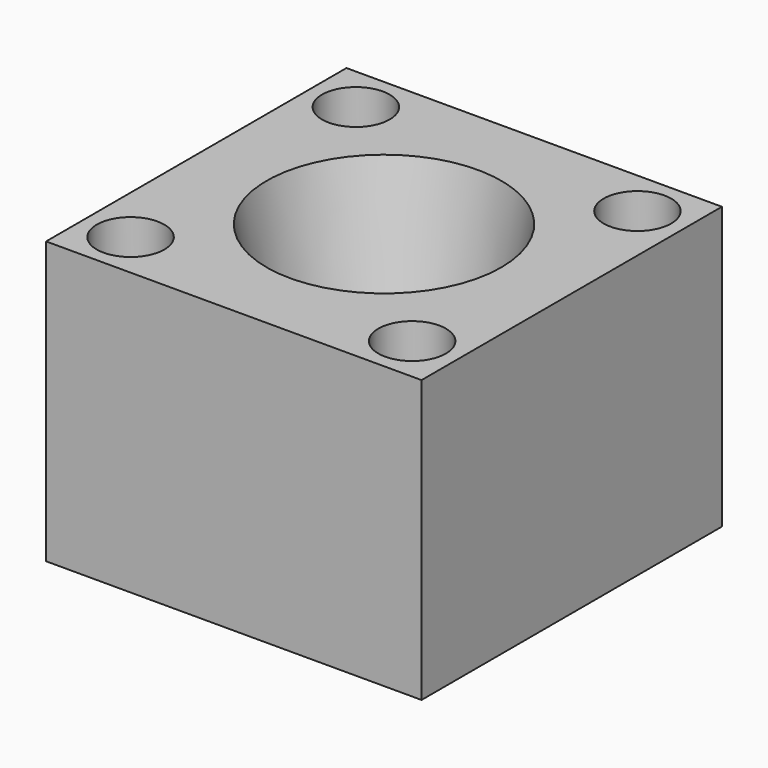
from build123d import *

# Parameters (mm, degrees)
F0_W             = 50.8
F0_H             = 50.8
F1_DEPTH         = 38.1
F2_R             = 15.875
F4_R             = 9.525
F6_R             = 4.572
F7_DEPTH         = 25.4
F9_R             = 2.286
F10_DEPTH        = 12.701
F10_COPIES_COUNT = 4


# Not quite as in the source:
# - a pattern or mirror of a feature is missing from the dataset's text; its kind, count and spacing are read off the source's solid


with BuildPart() as f1:
    # F0 (on Top) → F1 (new body)
    with BuildSketch(Plane.XY):
        Rectangle(F0_W, F0_H)
    extrude(amount=F1_DEPTH)

    # F2 (on face) → F5 section 0
    with BuildSketch(Plane.XY.offset(38.1)):
        Circle(F2_R)
    # F4 (on offset) → F5 section 1
    with BuildSketch(Plane(origin=(0, 0, 6.35), x_dir=(1, 0, 0), z_dir=(0, 0, -1))):
        Circle(F4_R)
    loft(mode=Mode.SUBTRACT)

    # F6 (on face) → F7 (cut)
    with BuildSketch(Plane.XY.offset(38.1)):
        with Locations((19.05, -19.05)):
            Circle(F6_R)
        with Locations((19.05, 19.05)):
            Circle(F6_R)
        with Locations((-19.05, 19.05)):
            Circle(F6_R)
        with Locations((-19.05, -19.05)):
            Circle(F6_R)
    extrude(amount=-F7_DEPTH, mode=Mode.SUBTRACT)

    # F9 (on offset) → F10 (cut, through all)
    with BuildSketch(Plane.XY.offset(12.7)):
        with Locations((-19.05, 19.05)):
            Circle(F9_R)
    f10 = extrude(amount=-F10_DEPTH, mode=Mode.SUBTRACT)

    # F10_copies: F10 ×4 about axis
    f10_copies_axis = Axis((0, 0, 0), (0, 0, 1))
    for i in range(1, F10_COPIES_COUNT):
        add(f10.rotate(f10_copies_axis, i * 360 / F10_COPIES_COUNT), mode=Mode.SUBTRACT)


solid = f1.part
